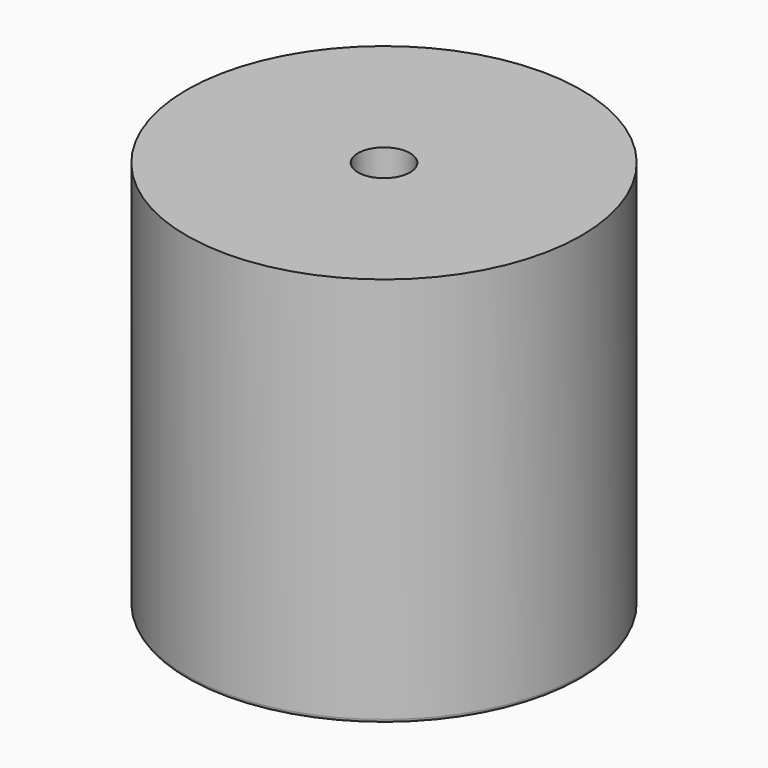
from build123d import *

# Parameters (mm, degrees)
F2_R = 0.2


with BuildPart() as f1:
    # F0 (on Front) → F1 (revolve)
    with BuildSketch(Plane.XZ):
        Polygon((1.4, 18), (7.6, 18), (7.6, 0), (10.6, 0), (10.6, 21), (1.4, 21), align=None)
    revolve(axis=Axis((0, 0, 19.3304718956), (0, 0, -1)))

    # F2
    f2_edges = [f1.edges().sort_by_distance(p)[0] for p in [
        (-7.6, 0, 0),
        (-10.6, 0, 0),
        (-7.6, 0, 18),
    ]]
    fillet(f2_edges, radius=F2_R)


solid = f1.part
